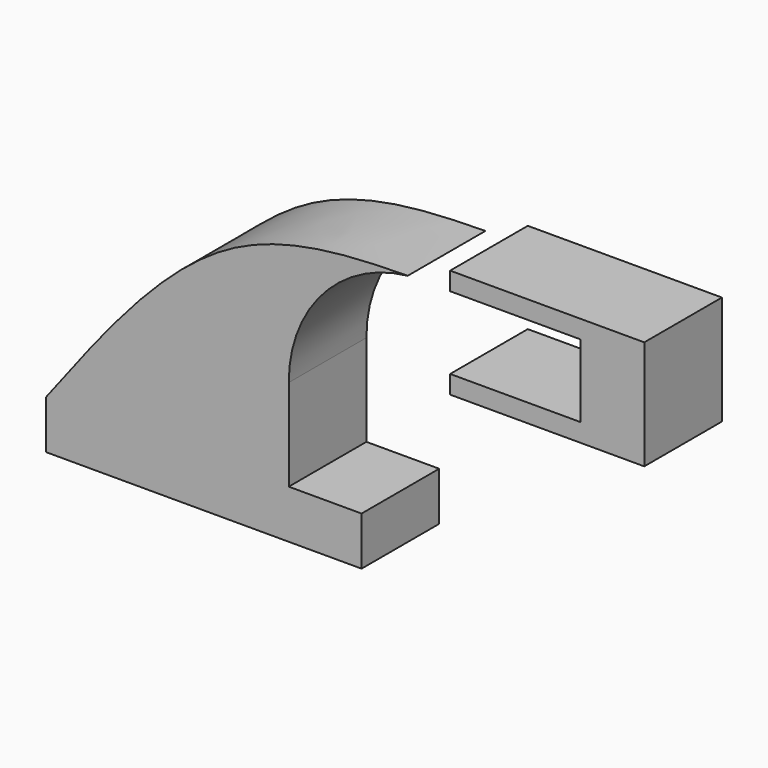
from build123d import *

# Parameters (mm, degrees)
F1_DEPTH = 25.4


with BuildPart() as f1:
    # F0 (on Front) → F1 (new body)
    with BuildSketch(Plane.XZ):
        Polygon((-41.275, -6.35), (41.275, -6.35), (41.275, 6.35), (22.225, 6.35), (-41.275, 6.35), align=None)
        with BuildLine():
            add(Edge.make_bspline(
                [(-41.275, 6.35), (-25.7957625049, 26.7914881612), (1.4845995339, 62.8172418731), (37.5652658057, 64.8833178289), (53.3598609175, 65.0570964203)],
                knots=[0, 0, 0, 0, 0.5376939005, 0.9476231808, 0.9476231808, 0.9476231808, 0.9476231808], degree=3))
            Line((-41.275, 6.35), (22.225, 6.35))
            Line((22.225, 6.35), (22.225, 30.3383627058))
            ThreePointArc((22.225, 30.3383627058), (31.1487862547, 53.6555775646), (53.3598609175, 65.0570964203))
        make_face()
    extrude(amount=F1_DEPTH)


with BuildPart() as f1b:
    # F0 (on Front) → F1, piece 2 (new body)
    with BuildSketch(Plane.XZ):
        Polygon((98.536185044, 46.0502), (64.4524941912, 46.0502), (64.4524941912, 41.275), (115.2524941912, 41.275), (115.2524941912, 69.85), (64.4524941912, 69.85), (64.4524941912, 65.1002), (98.536185044, 65.1002), align=None)
    extrude(amount=F1_DEPTH)


solid = Compound([f1.part, f1b.part])
